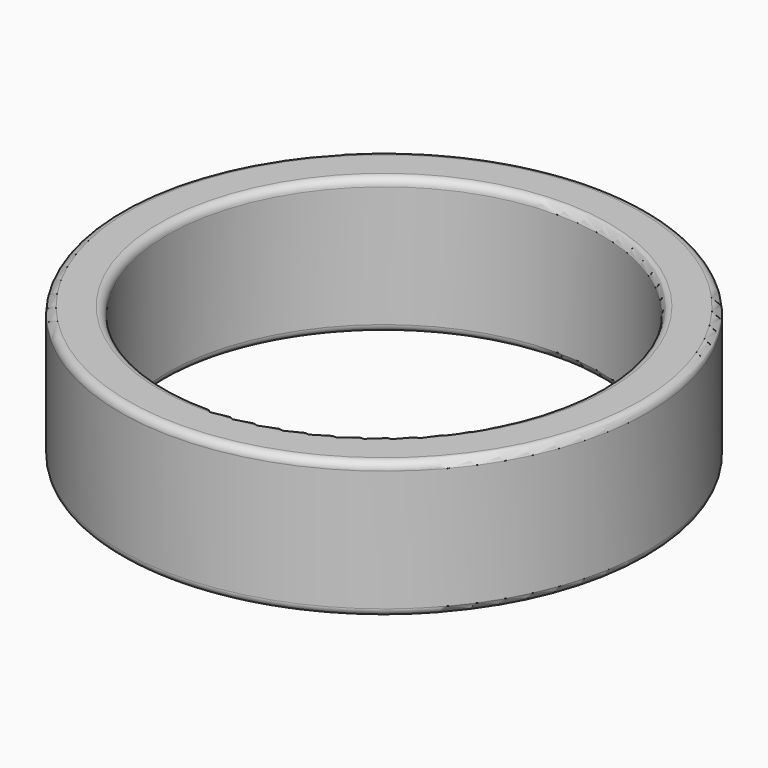
from build123d import *

# Parameters (mm, degrees)
F0_R     = 13.5
F0_R_2   = 11.1
F1_DEPTH = 7
F2_R     = 0.4


# Not quite as in the source:
# - a feature names something its author has since deleted; it is built from what else it names


with BuildPart() as f1:
    # F0 (on Top) → F1 (new body)
    with BuildSketch(Plane.XY):
        Circle(F0_R)
        Circle(F0_R_2, mode=Mode.SUBTRACT)
    extrude(amount=F1_DEPTH)

    # F2
    f2_edges = [f1.edges().sort_by_distance(p)[0] for p in [
        (-11.1, 0, 7),
        (-13.5, 0, 7),
        (-13.5, 0, 0),
        (-11.1, 0, 0),
    ]]
    fillet(f2_edges, radius=F2_R)


solid = f1.part
